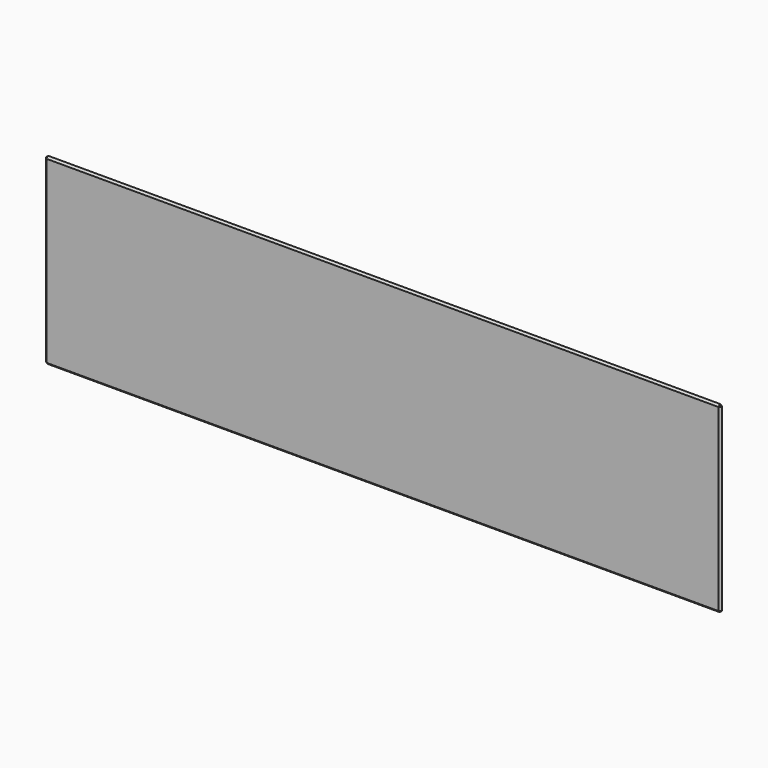
from build123d import *

# Parameters (mm, degrees)
F0_W     = 350
F0_H     = 95
F1_DEPTH = 2
F2_SIZE  = 0.99999


# Not quite as in the source:
# - a fillet or chamfer is up to 0.001 mm smaller than in the source, because OpenCascade refuses the exact size


with BuildPart() as f1:
    # F0 (on Front) → F1 (new body)
    with BuildSketch(Plane.XZ):
        Rectangle(F0_W, F0_H)
    extrude(amount=F1_DEPTH)

    # F2 (size 1 in the source; OpenCascade refuses exactly that, so slightly less here)
    f2_edges = [f1.edges().sort_by_distance(p)[0] for p in [
        (-175, -2, 0),
        (0, -2, 47.5),
        (0, -2, -47.5),
        (175, -2, 0),
        (-175, 0, 0),
        (0, 0, 47.5),
        (175, 0, 0),
        (0, 0, -47.5),
        (175, -1, -47.5),
        (175, -1, 47.5),
        (-175, -1, -47.5),
        (-175, -1, 47.5),
    ]]
    chamfer(f2_edges, length=F2_SIZE)


solid = f1.part
